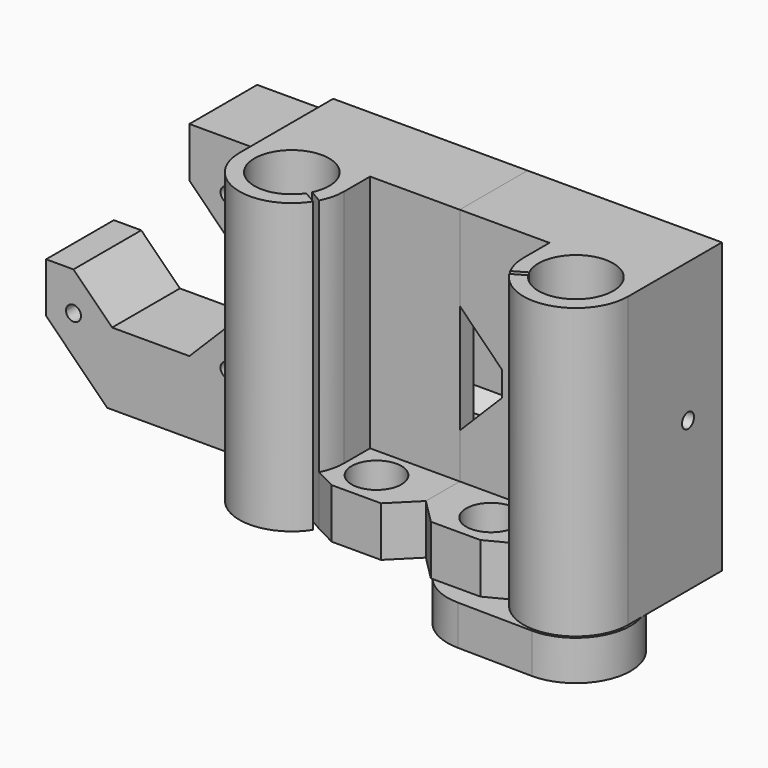
from build123d import *

# Parameters (mm, degrees)
F1_DEPTH  = 58
F3_R      = 5
F4_DEPTH  = 10
F5_SIZE   = 5
F2_R      = 4
F7_DEPTH  = 33
F8_R      = 1.5
F9_DEPTH  = 78.001
F10_DEPTH = 37
F11_R     = 1.5
F12_DEPTH = 17
F13_DEPTH = 40
F14_W     = 10
F14_H     = 22
F15_REACH = 67.1670919472
F17_DEPTH = 17.001
F18_R     = 2
F19_DEPTH = 8


with BuildPart() as f1:
    # F0 (on Top) → F1 (new body)
    with BuildSketch(Plane.XY):
        with BuildLine():
            Line((-10.5, 6.5), (-10.5, 0))
            ThreePointArc((-10.5, 0), (-10.2040674771, -2.4752791606), (-9.3329510623, -4.811031539))
            Line((-9.3329510623, -4.811031539), (-6.7307406984, -3.3086446849))
            ThreePointArc((-6.7307406984, -3.3086446849), (6.4951905284, 3.75), (-6.2307406984, -4.1746700887))
            Line((-6.2307406984, -4.1746700887), (-8.8329510623, -5.6770569427))
            ThreePointArc((-8.8329510623, -5.6770569427), (2.958379104, -10.0746212374), (10.5, 0))
            Line((10.5, 0), (10.5, 23.5))
            Line((10.5, 23.5), (-28.5, 23.5))
            Line((-28.5, 23.5), (-28.5, 6.5))
            Line((-28.5, 6.5), (-10.5, 6.5))
        make_face()
    extrude(amount=F1_DEPTH)

    # F3 (on Top) → F4 (join)
    with BuildSketch(Plane.XY):
        with BuildLine():
            Line((-10.5, 0), (-10.5, 6.5))
            Line((-10.5, 6.5), (-28.5, 6.5))
            Line((-28.5, 6.5), (-28.5, -7))
            Line((-28.5, -7), (-13.5793450754, -7))
            Line((-13.5793450754, -7), (-9.3329510623, -4.811031539))
            ThreePointArc((-9.3329510623, -4.811031539), (-10.2040674771, -2.4752791606), (-10.5, 0))
        make_face()
        with Locations((-17, 0)):
            Circle(F3_R, mode=Mode.SUBTRACT)
    extrude(amount=F4_DEPTH)

    # F5
    f5_edges = [f1.edges().sort_by_distance(p)[0] for p in [
        (-28.5, -7, 5),
    ]]
    chamfer(f5_edges, length=F5_SIZE)


with BuildPart() as f6_1:
    # F6: instance of F1
    add(f1.part.mirror(Plane(origin=(-28.5, 13.9880952381, 27.0952380952), x_dir=(0, -1, 0), z_dir=(-1, 0, 0))))


with BuildPart() as f1_1:
    add(f1.part)

    # F2 (on face) → F7 (cut)
    with BuildSketch(Plane(origin=(-28.5, 0, 0), x_dir=(0, -1, 0), z_dir=(-1, 0, 0))):
        Polygon((-17, 44), (-20, 41), (-20, 19), (-17, 16), (-13, 16), (-10, 19), (-10, 41), (-13, 44), align=None)
        with Locations((-15, 6.5)):
            Circle(F2_R)
        with Locations((-15, 51.5)):
            Circle(F2_R)
    extrude(amount=-F7_DEPTH, mode=Mode.SUBTRACT)


with BuildPart() as f9_tool:
    # F8 (on face) → F9 (new body, through all)
    with BuildSketch(Plane.YZ.offset(10.5)):
        with Locations((15, 30)):
            Circle(F8_R)
    extrude(amount=-F9_DEPTH)


with BuildPart() as f1_2:
    add(f1_1.part)

    # F9: cut by f9_tool
    add(f9_tool.part, mode=Mode.SUBTRACT)

    # F16 (on face) → F17 (cut, through all)
    with BuildSketch(Plane.XZ.offset(-6.5)):
        Polygon((-20.029462827, 32.5), (-28.5, 41), (-28.5, 19), (-20.029462827, 27.5), align=None)
    extrude(amount=-F17_DEPTH, mode=Mode.SUBTRACT)


with BuildPart() as f6_1_1:
    add(f6_1.part)

    # F9: cut by f9_tool
    add(f9_tool.part, mode=Mode.SUBTRACT)

    # F2 (on face) → F10 (cut)
    with BuildSketch(Plane(origin=(-28.5, 0, 0), x_dir=(0, -1, 0), z_dir=(-1, 0, 0))):
        with Locations((-15, 51.5)):
            Circle(F2_R)
        with Locations((-15, 6.5)):
            Circle(F2_R)
    extrude(amount=F10_DEPTH, mode=Mode.SUBTRACT)

    # F11 (on face) → F12 (join)
    with BuildSketch(Plane(origin=(0, 23.5, 0), x_dir=(-1, 0, 0), z_dir=(0, 1, 0))):
        Polygon((67.5, 55.5), (67.5, 0), (99.25, 0), (111.5, 12.25), (111.5, 22.25), (106, 22.25), (102.125, 18.375), (98.25, 14.5), (82.75, 14.5), (75, 22.25), (75, 37.75), (82.75, 45.5), (82.75, 55.5), align=None)
        with Locations((75, 14.5)):
            Circle(F11_R, mode=Mode.SUBTRACT)
        with BuildLine():
            ThreePointArc((107.5, 14.5), (105.4259748515, 13.1141807012), (104.9393398282, 15.5606601718))
            ThreePointArc((104.9393398282, 15.5606601718), (106.5740251485, 15.8858192988), (107.5, 14.5))
        make_face(mode=Mode.SUBTRACT)
        with Locations((75, 45.5)):
            Circle(F11_R, mode=Mode.SUBTRACT)
    extrude(amount=-F12_DEPTH)

    # F2 (on face) → F13 (cut)
    with BuildSketch(Plane(origin=(-28.5, 0, 0), x_dir=(0, -1, 0), z_dir=(-1, 0, 0))):
        Polygon((-17, 44), (-20, 41), (-20, 19), (-17, 16), (-13, 16), (-10, 19), (-10, 41), (-13, 44), align=None)
    extrude(amount=F13_DEPTH, mode=Mode.SUBTRACT)

    f15_end = Plane(origin=(-102.125, 15, 18.375), x_dir=(0.7071067812, 0, -0.7071067812), z_dir=(0.7071067812, 0, 0.7071067812))
    # F14 (on face) → F15 (cut, up to a plane its end follows)
    with BuildSketch(Plane.YZ.offset(-68.5)):
        with Locations((15, 30)):
            Rectangle(F14_W, F14_H)
    f15_long = extrude(amount=-F15_REACH, mode=Mode.PRIVATE)
    add(split(f15_long, bisect_by=f15_end, keep=Keep.TOP, mode=Mode.PRIVATE), mode=Mode.SUBTRACT)


with BuildPart() as f19:
    # F18 (on Top) → F19 (new body)
    with BuildSketch(Plane.XY):
        with BuildLine():
            ThreePointArc((-15, 4), (-11, 0), (-15, -4))
            Line((-15, -4), (-25, -4))
            ThreePointArc((-25, -4), (-21.0381570675, -8.9185570149), (-15, -10.7703296143))
            Line((-15, -10.7703296143), (0, -11))
            ThreePointArc((0, -11), (11, 0), (0, 11))
            Line((0, 11), (-15, 10.7703296143))
            ThreePointArc((-15, 10.7703296143), (-21.0381570675, 8.9185570149), (-25, 4))
            Line((-25, 4), (-15, 4))
        make_face()
        with Locations((0, -8)):
            Circle(F18_R, mode=Mode.SUBTRACT)
        with Locations((-8, 0)):
            Circle(F18_R, mode=Mode.SUBTRACT)
        with BuildLine():
            ThreePointArc((0, 5), (5, 0), (0, -5))
            ThreePointArc((0, -5), (-5, 0), (0, 5))
        make_face(mode=Mode.SUBTRACT)
        with Locations((8, 0)):
            Circle(F18_R, mode=Mode.SUBTRACT)
        with Locations((0, 8)):
            Circle(F18_R, mode=Mode.SUBTRACT)
    extrude(amount=-F19_DEPTH)


solid = Compound([f1_2.part, f6_1_1.part, f19.part])
